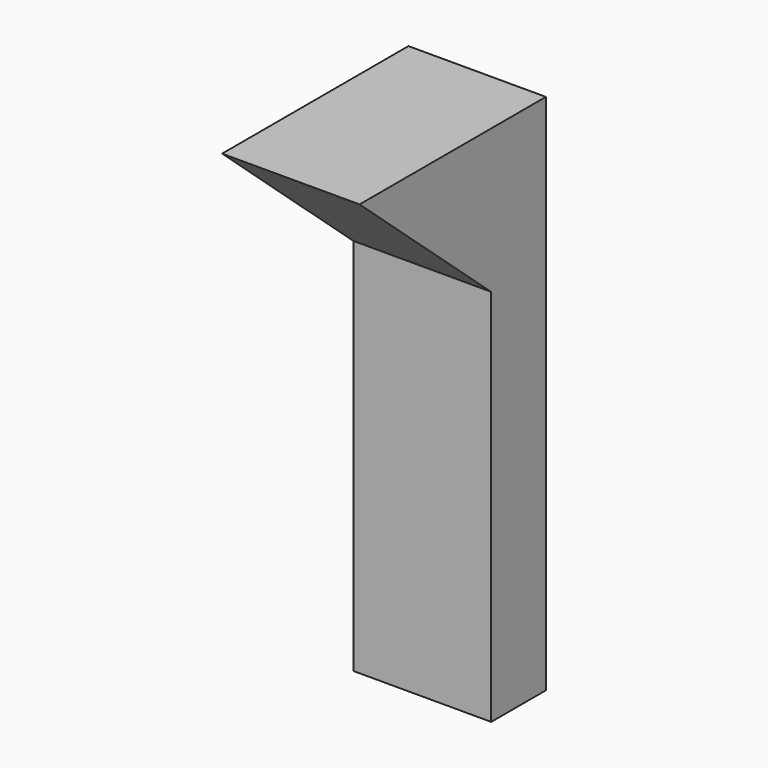
from build123d import *

# Parameters (mm, degrees)
F0_W        = 51.0822050273
F0_H        = 117.4111329019
F1_DEPTH    = 25.4
F2_DEPTH    = 76.7365470529
F3_W        = 51.0822050273
F3_H        = 53.3235035837
F4_DEPTH    = 61.1563976854
F5_T1_DEPTH = 365.1602492866


# Not quite as in the source:
# - a fillet or chamfer that OpenCascade refuses, or shapes differently, is made with other operations: its cross-section is extruded or revolved along the edge and cut away or added


with BuildPart() as f1:
    # F0 (on Front) → F1 (new body)
    with BuildSketch(Plane.XZ):
        with Locations((-25.5411025137, 1.6260724515)):
            Rectangle(F0_W, F0_H)
    extrude(amount=F1_DEPTH)

    # F2 (add): a face of the model
    f2_faces = [f1.faces().sort_by_distance(p)[0] for p in [
        (-25.5411025137, -12.7, 60.3316389024),
    ]]
    extrude(f2_faces, amount=F2_DEPTH)

    # F3 (on face) → F4 (join)
    with BuildSketch(Plane.XZ.offset(25.4)):
        with Locations((-25.5411025137, 110.4064341635)):
            Rectangle(F3_W, F3_H)
    extrude(amount=F4_DEPTH)

    # F5: chamfer of 60.96 x 53.34 on 1 edges, made by hand

    # F5_s2 → F5_t1 (cut)
    with BuildSketch(Plane.YZ.offset(-208.121227157)):
        Polygon((-25.5963976854, 83.7446823716), (-86.5563976854, 137.0846823716), (-86.5563976854, 83.7446823716), align=None)
    extrude(amount=F5_T1_DEPTH, mode=Mode.SUBTRACT)


solid = f1.part
